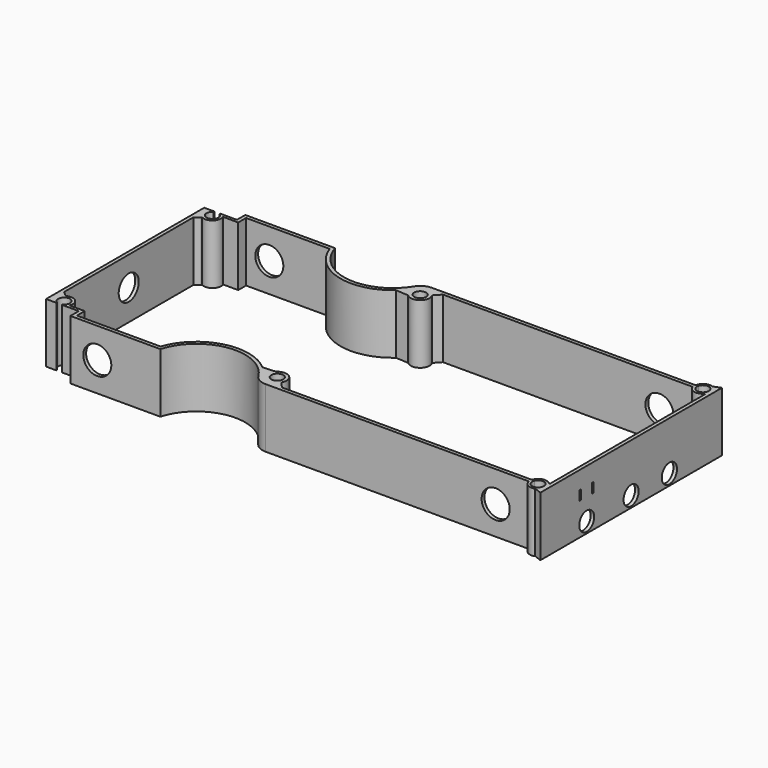
from build123d import *

# Parameters (mm, degrees)
F0_R     = 2
F1_DEPTH = 20
F2_R     = 4.7152449582
F2_R_2   = 4.7232891339
F3_DEPTH = 108
F4_R     = 4.2098088582
F5_DEPTH = 25
F6_R     = 3.1711780618
F6_R_2   = 3.2066806009
F6_R_3   = 3.1312270379
F6_W     = 0.6074849516
F6_H     = 3.2243365422
F6_W_2   = 0.6542131305
F7_DEPTH = 25


# Not quite as in the source:
# - a feature names something its author has since deleted; it is built from what else it names


with BuildPart() as f1:
    # F0 (on Top) → F1 (new body)
    with BuildSketch(Plane.XY):
        with BuildLine():
            Line((-164.65269916, 33.20941329), (-164.65269916, 32.9194632454))
            ThreePointArc((-164.65269916, 32.9194632454), (-165.5739976736, 29.1538786951), (-166.563206189, 32.902196247))
            Line((-166.563206189, 32.902196247), (-166.563206189, 33.20941329))
            Line((-166.563206189, 33.20941329), (-170, 33.20941329))
            Line((-170, 33.20941329), (-170, 0))
            Line((-170, 0), (-170, -33.20941329))
            Line((-170, -33.20941329), (-166.563206189, -33.20941329))
            Line((-166.563206189, -33.20941329), (-166.563206189, -32.902196247))
            ThreePointArc((-166.563206189, -32.902196247), (-165.5739976736, -29.1538786951), (-164.65269916, -32.9194632454))
            Line((-164.65269916, -32.9194632454), (-164.65269916, -33.20941329))
            Line((-164.65269916, -33.20941329), (-163.2265451578, -33.20941329))
            Line((-163.2265451578, -33.20941329), (-159.009280774, -33.20941329))
            Line((-159.009280774, -33.20941329), (-159.009280774, -36.7204154693))
            Line((-159.009280774, -36.7204154693), (-157.7970415085, -36.7204154693))
            Line((-157.7970415085, -36.7204154693), (-128.8103089121, -36.7204154693))
            ThreePointArc((-128.8103089121, -36.7204154693), (-115.3036395578, -25.0214683637), (-99.1359348061, -32.6307261124))
            ThreePointArc((-99.1359348061, -32.6307261124), (-97.3177205123, -34.3677013727), (-94.8839611325, -35))
            Line((-94.8839611325, -35), (-6.3253850676, -35))
            ThreePointArc((-6.3253850676, -35), (-4.9357568901, -37.0403297798), (-2.4707801799, -37.1741277646))
            Line((-2.4707801799, -37.1741277646), (0, -38.1401939384))
            Line((0, -38.1401939384), (0, -35))
            Line((0, -35), (0, 0))
            Line((0, 0), (0, 35))
            Line((0, 35), (0, 38.1401939384))
            Line((0, 38.1401939384), (-2.4707801799, 37.1741277646))
            ThreePointArc((-2.4707801799, 37.1741277646), (-4.9357568901, 37.0403297798), (-6.3253850676, 35))
            Line((-6.3253850676, 35), (-94.8839611325, 35))
            ThreePointArc((-94.8839611325, 35), (-97.3177205123, 34.3677013727), (-99.1359348061, 32.6307261124))
            ThreePointArc((-99.1359348061, 32.6307261124), (-115.3036395578, 25.0214683637), (-128.8103089121, 36.7204154693))
            Line((-128.8103089121, 36.7204154693), (-157.7970415085, 36.7204154693))
            Line((-157.7970415085, 36.7204154693), (-159.009280774, 36.7204154693))
            Line((-159.009280774, 36.7204154693), (-159.009280774, 33.20941329))
            Line((-159.009280774, 33.20941329), (-163.2265451578, 33.20941329))
            Line((-163.2265451578, 33.20941329), (-164.65269916, 33.20941329))
        make_face()
        with Locations((-94.8839611325, -30)):
            Circle(F0_R, mode=Mode.SUBTRACT)
        with BuildLine():
            ThreePointArc((-1.5680128924, -34.6153974533), (-1.5847981725, -34.8739692511), (-1.6348722671, -35.1282008489))
            ThreePointArc((-1.6348722671, -35.1282008489), (-3.5680128924, -36.6153974533), (-5.5011535178, -35.1282008489))
            ThreePointArc((-5.5011535178, -35.1282008489), (-5.561565475, -34.4549353061), (-5.3942458987, -33.8))
            ThreePointArc((-5.3942458987, -33.8), (-3.5680128924, -32.6153974533), (-1.7417798862, -33.8))
            ThreePointArc((-1.7417798862, -33.8), (-1.6119369721, -34.1985437695), (-1.5680128924, -34.6153974533))
        make_face(mode=Mode.SUBTRACT)
        with Locations((-94.8839611325, 30)):
            Circle(F0_R, mode=Mode.SUBTRACT)
        with BuildLine():
            Line((-1.5434729926, 32.5735324938), (-1.2, 32.5194895267))
            Line((-1.2, 32.5194895267), (-1.2, 0))
            Line((-1.2, 0), (-1.2, -32.5194895267))
            Line((-1.2, -32.5194895267), (-1.5434729926, -32.5735324938))
            ThreePointArc((-1.5434729926, -32.5735324938), (-4.2823772406, -31.8301402125), (-6.3253850676, -33.8))
            Line((-6.3253850676, -33.8), (-90.2593984932, -33.8))
            Line((-90.2593984932, -33.8), (-92.2271985619, -31.6787384118))
            ThreePointArc((-92.2271985619, -31.6787384118), (-92.912700117, -27.5524134293), (-97.0903228742, -27.7620281778))
            Line((-97.0903228742, -27.7620281778), (-101.4582490544, -28.045448372))
            ThreePointArc((-101.4582490544, -28.045448372), (-117.5672901619, -24.2537650751), (-129.6891982841, -35.5204154693))
            Line((-129.6891982841, -35.5204154693), (-155.884909603, -35.5204154693))
            Line((-155.884909603, -35.5204154693), (-157.7970415085, -35.5204154693))
            Line((-157.7970415085, -35.5204154693), (-157.7970415085, -32.2268303811))
            Line((-157.7970415085, -32.2268303811), (-162.8932879486, -32.2268303811))
            ThreePointArc((-162.8932879486, -32.2268303811), (-163.6774302758, -28.9699966079), (-167.0088434251, -28.6185256358))
            Line((-167.0088434251, -28.6185256358), (-167.2241950518, -28.4767444108))
            Line((-167.2241950518, -28.4767444108), (-168.8, -27.1884445101))
            Line((-168.8, -27.1884445101), (-168.8, 0))
            Line((-168.8, 0), (-168.8, 27.1884445101))
            Line((-168.8, 27.1884445101), (-167.2241950518, 28.4767444108))
            Line((-167.2241950518, 28.4767444108), (-167.0088434251, 28.6185256358))
            ThreePointArc((-167.0088434251, 28.6185256358), (-163.6774302758, 28.9699966079), (-162.8932879486, 32.2268303811))
            Line((-162.8932879486, 32.2268303811), (-157.7970415085, 32.2268303811))
            Line((-157.7970415085, 32.2268303811), (-157.7970415085, 35.5204154693))
            Line((-157.7970415085, 35.5204154693), (-155.884909603, 35.5204154693))
            Line((-155.884909603, 35.5204154693), (-129.6891982841, 35.5204154693))
            ThreePointArc((-129.6891982841, 35.5204154693), (-117.5672901619, 24.2537650751), (-101.4582490544, 28.045448372))
            Line((-101.4582490544, 28.045448372), (-97.0903228742, 27.7620281778))
            ThreePointArc((-97.0903228742, 27.7620281778), (-92.912700117, 27.5524134293), (-92.2271985619, 31.6787384118))
            Line((-92.2271985619, 31.6787384118), (-90.2593984932, 33.8))
            Line((-90.2593984932, 33.8), (-6.3253850676, 33.8))
            ThreePointArc((-6.3253850676, 33.8), (-4.2823772406, 31.8301402125), (-1.5434729926, 32.5735324938))
        make_face(mode=Mode.SUBTRACT)
        with BuildLine():
            ThreePointArc((-1.7417798862, 33.8), (-3.5680128924, 32.6153974533), (-5.3942458987, 33.8))
            ThreePointArc((-5.3942458987, 33.8), (-5.561565475, 34.4549353061), (-5.5011535178, 35.1282008489))
            ThreePointArc((-5.5011535178, 35.1282008489), (-3.5680128924, 36.6153974533), (-1.6348722671, 35.1282008489))
            ThreePointArc((-1.6348722671, 35.1282008489), (-1.5847981725, 34.8739692511), (-1.5680128924, 34.6153974533))
            ThreePointArc((-1.5680128924, 34.6153974533), (-1.6119369721, 34.1985437695), (-1.7417798862, 33.8))
        make_face(mode=Mode.SUBTRACT)
    extrude(amount=F1_DEPTH)

    # F2 (on face) → F3 (cut)
    with BuildSketch(Plane.XZ.offset(36.7204154693)):
        with Locations((-149.9848365784, 9.8437862471)):
            Circle(F2_R)
        with Locations((-17.5157543272, 9.6355015412)):
            Circle(F2_R_2)
    extrude(amount=-F3_DEPTH, mode=Mode.SUBTRACT)

    # F4 (on face) → F5 (cut)
    with BuildSketch(Plane(origin=(-170, 0, 0), x_dir=(0, -1, 0), z_dir=(-1, 0, 0))):
        with Locations((0, 10.2570122108)):
            Circle(F4_R)
    extrude(amount=-F5_DEPTH, mode=Mode.SUBTRACT)

    # F6 (on face) → F7 (cut)
    with BuildSketch(Plane.YZ):
        with Locations((0, 3.6681490019)):
            Circle(F6_R)
        with Locations((16.0749554634, 3.6681490019)):
            Circle(F6_R_2)
        with Locations((-18.6450798064, 3.6681490019)):
            Circle(F6_R_3)
        with Locations((-21.4254865423, 12.4766645022)):
            Rectangle(F6_W, F6_H)
        with Locations((-16.1684155464, 12.4766645022)):
            Rectangle(F6_W_2, F6_H)
    extrude(amount=-F7_DEPTH, mode=Mode.SUBTRACT)


solid = f1.part
